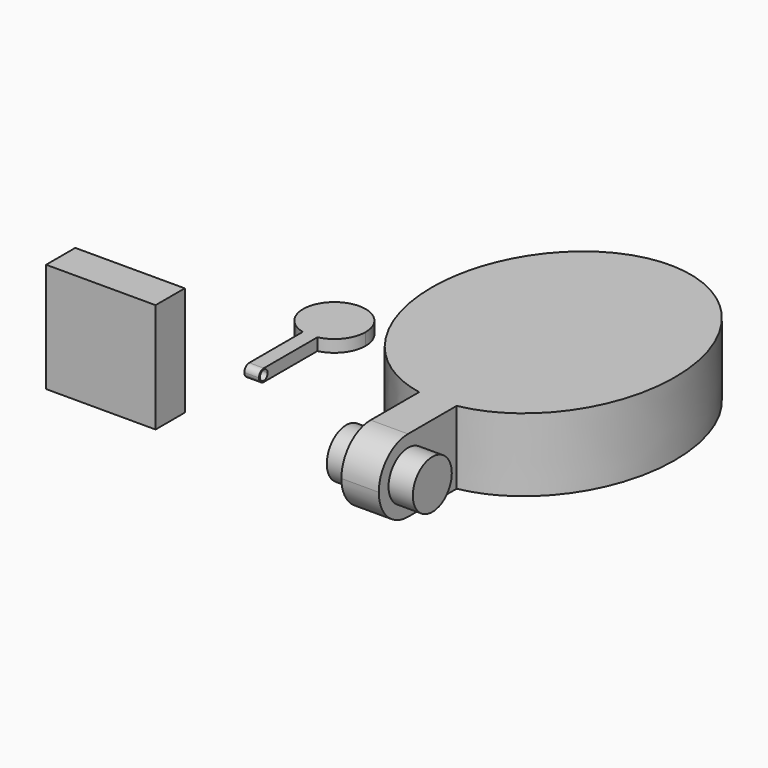
from build123d import *

# Parameters (mm, degrees)
F1_DEPTH  = 5
F2_DEPTH  = 5
F4_DEPTH  = 10
F6_DEPTH  = 5
F8_DEPTH  = 20
F10_DEPTH = 20
F11_R     = 2.5
F12_R     = 2.49999
F13_W     = 6.5
F13_H     = 45
F14_DEPTH = 5
F15_W     = 3
F15_H     = 5
F16_DEPTH = 5
F17_R     = 2
F18_DEPTH = 3
F19_R     = 2
F20_DEPTH = 3
F22_DEPTH = 30
F23_DEPTH = 30
F25_DEPTH = 10
F26_R     = 10
F27_DEPTH = 10
F28_R     = 15
F29_R     = 14.99999


# Not quite as in the source:
# - a fillet or chamfer is up to 0.001 mm smaller than in the source, because OpenCascade refuses the exact size


with BuildPart() as f1:
    # F0 (on Top) → F1 (new body)
    with BuildSketch(Plane.XY):
        with BuildLine():
            ThreePointArc((0, -12.5), (8.8388347648, -8.8388347648), (12.5, 0))
            ThreePointArc((12.5, 0), (-8.8388347648, 8.8388347648), (0, -12.5))
        make_face()
    extrude(amount=F1_DEPTH)

    # F0 (on Top) → F2 (join)
    with BuildSketch(Plane.XY):
        with BuildLine():
            Line((-3, -12.5), (0, -12.5))
            Line((0, -12.5), (3, -12.5))
            ThreePointArc((3, -12.5), (10.0949215053, -7.9588039178), (12.8549601322, 0))
            ThreePointArc((12.8549601322, 0), (-7.9588039178, 10.0949215053), (-3, -12.5))
        make_face()
        with BuildLine():
            ThreePointArc((0, -12.5), (-8.8388347648, 8.8388347648), (12.5, 0))
            ThreePointArc((12.5, 0), (8.8388347648, -8.8388347648), (0, -12.5))
        make_face(mode=Mode.SUBTRACT)
        with BuildLine():
            Line((3, -12.5), (0, -12.5))
            Line((0, -12.5), (-3, -12.5))
            ThreePointArc((-3, -12.5), (0, -12.8549601322), (3, -12.5))
        make_face()
        with BuildLine():
            ThreePointArc((3, -12.5), (0, -12.8549601322), (-3, -12.5))
            Line((-3, -12.5), (-3, -42.5))
            Line((-3, -42.5), (3, -42.5))
            Line((3, -42.5), (3, -12.5))
        make_face()
    extrude(amount=F2_DEPTH)

    # F3 (on face) → F4 (cut)
    with BuildSketch(Plane.YZ.offset(3)):
        with BuildLine():
            ThreePointArc((-40, 4.5), (-41.4142135624, 3.9142135624), (-42, 2.5))
            Line((-42, 2.5), (-40, 2.5))
            Line((-40, 2.5), (-40, 4.5))
        make_face()
        with BuildLine():
            Line((-40, 2.5), (-42, 2.5))
            ThreePointArc((-42, 2.5), (-40, 0.5), (-38, 2.5))
            ThreePointArc((-38, 2.5), (-38.5857864376, 3.9142135624), (-40, 4.5))
            Line((-40, 4.5), (-40, 2.5))
        make_face()
    extrude(amount=-F4_DEPTH, mode=Mode.SUBTRACT)

    # F11
    f11_edges = [f1.edges().sort_by_distance(p)[0] for p in [
        (0, -42.5, 5),
    ]]
    fillet(f11_edges, radius=F11_R)

    # F12 (radius 2.5 in the source; OpenCascade refuses exactly that, so slightly less here)
    f12_edges = [f1.edges().sort_by_distance(p)[0] for p in [
        (0, -42.5, 0),
    ]]
    fillet(f12_edges, radius=F12_R)


with BuildPart() as f6:
    # F5 (on Top) → F6 (new body)
    with BuildSketch(Plane.XY):
        Polygon((-46.75, -47.5), (-50, -47.5), (-53.25, -47.5), (-53.25, -42.5), (-72.5, -42.5), (-72.5, -57.5), (-27.5, -57.5), (-27.5, -42.5), (-46.75, -42.5), align=None)
    extrude(amount=F6_DEPTH)

    # F7 (on face) → F8 (join)
    with BuildSketch(Plane.XY.offset(5)):
        Polygon((-53.25, -42.5), (-72.5, -42.5), (-72.5, -57.5), (-27.5, -57.5), (-27.5, -42.5), (-46.75, -42.5), (-46.75, -47.5), (-53.25, -47.5), align=None)
    extrude(amount=F8_DEPTH)

    # F9 (on face) → F10 (join)
    with BuildSketch(Plane(origin=(0, 0, 0), x_dir=(1, 0, 0), z_dir=(0, 0, -1))):
        Polygon((-46.75, 42.5), (-27.5, 42.5), (-27.5, 57.5), (-72.5, 57.5), (-72.5, 42.5), (-53.25, 42.5), (-53.25, 47.5), (-46.75, 47.5), align=None)
    extrude(amount=F10_DEPTH)

    # F13 (on face) → F14 (join)
    with BuildSketch(Plane(origin=(0, -47.5, 0), x_dir=(-1, 0, 0), z_dir=(0, 1, 0))):
        with Locations((50, 2.5)):
            Rectangle(F13_W, F13_H)
    extrude(amount=F14_DEPTH)

    # F15 (on face) → F16 (join)
    with BuildSketch(Plane(origin=(0, -42.5, 0), x_dir=(-1, 0, 0), z_dir=(0, 1, 0))):
        with Locations((54.5, 2.5)):
            Rectangle(F15_W, F15_H)
        with Locations((45.5, 2.5)):
            Rectangle(F15_W, F15_H)
    extrude(amount=F16_DEPTH)

    # F17 (on face) → F18 (cut)
    with BuildSketch(Plane(origin=(-56, 0, 0), x_dir=(0, -1, 0), z_dir=(-1, 0, 0))):
        with Locations((40, 2.5)):
            Circle(F17_R)
    extrude(amount=-F18_DEPTH, mode=Mode.SUBTRACT)

    # F19 (on face) → F20 (cut)
    with BuildSketch(Plane.YZ.offset(-44)):
        with Locations((-40, 2.5)):
            Circle(F19_R)
    extrude(amount=-F20_DEPTH, mode=Mode.SUBTRACT)


with BuildPart() as f22:
    # F21 (on Top) → F22 (new body)
    with BuildSketch(Plane.XY):
        with BuildLine():
            add(Edge.make_bspline(
                [(90, -60), (93.8671431109, -60), (97.6882954661, -59.2864382677)],
                knots=[0, 0, 0, 0.1543783876, 0.1543783876, 0.1543783876], degree=2, weights=[1, 0.997022393, 1]))
            Line((97.6882954661, -59.2864382677), (90, -59.2864382677))
            Line((90, -59.2864382677), (90, -60))
        make_face()
        with BuildLine():
            add(Edge.make_bspline(
                [(97.6882954661, -59.2864382677), (205.0474477085, -39.2381974411), (122.5237238542, 45.5716867888), (40, 130.3815710188), (40, 0)],
                knots=[0.1543783876, 0.1543783876, 0.1543783876, 2.433383684, 2.433383684, 4.7123889804, 4.7123889804, 4.7123889804], degree=2, weights=[1, 0.4180463628, 1, 0.4180463628, 1]))
            Line((40, 0), (90, 0))
            Line((90, 0), (90, -59.2864382677))
            Line((90, -59.2864382677), (97.6882954661, -59.2864382677))
        make_face()
        with BuildLine():
            Line((90, 0), (40, 0))
            add(Edge.make_bspline(
                [(40, 0), (40, -51.3851534255), (82.3117045339, -59.2864382677)],
                knots=[4.7123889804, 4.7123889804, 4.7123889804, 6.1288069195, 6.1288069195, 6.1288069195], degree=2, weights=[1, 0.7595281131, 1]))
            Line((82.3117045339, -59.2864382677), (90, -59.2864382677))
            Line((90, -59.2864382677), (90, 0))
        make_face()
        with BuildLine():
            Line((90, -59.2864382677), (82.3117045339, -59.2864382677))
            add(Edge.make_bspline(
                [(82.3117045339, -59.2864382677), (86.1328568891, -60), (90, -60)],
                knots=[6.1288069195, 6.1288069195, 6.1288069195, 6.2831853072, 6.2831853072, 6.2831853072], degree=2, weights=[1, 0.997022393, 1]))
            Line((90, -60), (90, -59.2864382677))
        make_face()
    extrude(amount=F22_DEPTH)

    # F21 (on Top) → F23 (join)
    with BuildSketch(Plane.XY):
        with BuildLine():
            add(Edge.make_bspline(
                [(97.6882954661, -59.2864382677), (205.0474477085, -39.2381974411), (122.5237238542, 45.5716867888), (40, 130.3815710188), (40, 0)],
                knots=[0.1543783876, 0.1543783876, 0.1543783876, 2.433383684, 2.433383684, 4.7123889804, 4.7123889804, 4.7123889804], degree=2, weights=[1, 0.4180463628, 1, 0.4180463628, 1]))
            Line((40, 0), (90, 0))
            Line((90, 0), (90, -59.2864382677))
            Line((90, -59.2864382677), (97.6882954661, -59.2864382677))
        make_face()
        with BuildLine():
            Line((90, 0), (40, 0))
            add(Edge.make_bspline(
                [(40, 0), (40, -51.3851534255), (82.3117045339, -59.2864382677)],
                knots=[4.7123889804, 4.7123889804, 4.7123889804, 6.1288069195, 6.1288069195, 6.1288069195], degree=2, weights=[1, 0.7595281131, 1]))
            Line((82.3117045339, -59.2864382677), (90, -59.2864382677))
            Line((90, -59.2864382677), (90, 0))
        make_face()
        with BuildLine():
            Line((97.6882954661, -99.2864382677), (97.6882954661, -59.2864382677))
            add(Edge.make_bspline(
                [(90, -60), (93.8671431109, -60), (97.6882954661, -59.2864382677)],
                knots=[0, 0, 0, 0.1543783876, 0.1543783876, 0.1543783876], degree=2, weights=[1, 0.997022393, 1]))
            add(Edge.make_bspline(
                [(82.3117045339, -59.2864382677), (86.1328568891, -60), (90, -60)],
                knots=[6.1288069195, 6.1288069195, 6.1288069195, 6.2831853072, 6.2831853072, 6.2831853072], degree=2, weights=[1, 0.997022393, 1]))
            Line((82.3117045339, -59.2864382677), (82.3117045339, -99.2864382677))
            Line((82.3117045339, -99.2864382677), (97.6882954661, -99.2864382677))
        make_face()
        with BuildLine():
            add(Edge.make_bspline(
                [(90, -60), (93.8671431109, -60), (97.6882954661, -59.2864382677)],
                knots=[0, 0, 0, 0.1543783876, 0.1543783876, 0.1543783876], degree=2, weights=[1, 0.997022393, 1]))
            Line((97.6882954661, -59.2864382677), (90, -59.2864382677))
            Line((90, -59.2864382677), (90, -60))
        make_face()
        with BuildLine():
            Line((90, -59.2864382677), (82.3117045339, -59.2864382677))
            add(Edge.make_bspline(
                [(82.3117045339, -59.2864382677), (86.1328568891, -60), (90, -60)],
                knots=[6.1288069195, 6.1288069195, 6.1288069195, 6.2831853072, 6.2831853072, 6.2831853072], degree=2, weights=[1, 0.997022393, 1]))
            Line((90, -60), (90, -59.2864382677))
        make_face()
    extrude(amount=F23_DEPTH)

    # F24 (on face) → F25 (join)
    with BuildSketch(Plane.YZ.offset(97.6882954661)):
        with BuildLine():
            ThreePointArc((-94.2864382677, 15), (-84.2864382677, 5), (-74.2864382677, 15))
            ThreePointArc((-74.2864382677, 15), (-84.2864382677, 25), (-94.2864382677, 15))
        make_face()
    extrude(amount=F25_DEPTH)

    # F26 (on face) → F27 (join)
    with BuildSketch(Plane(origin=(82.3117045339, 0, 0), x_dir=(0, -1, 0), z_dir=(-1, 0, 0))):
        with Locations((84.2864382677, 15)):
            Circle(F26_R)
    extrude(amount=F27_DEPTH)

    # F28
    f28_edges = [f22.edges().sort_by_distance(p)[0] for p in [
        (90, -99.286438, 30),
    ]]
    fillet(f28_edges, radius=F28_R)

    # F29 (radius 15 in the source; OpenCascade refuses exactly that, so slightly less here)
    f29_edges = [f22.edges().sort_by_distance(p)[0] for p in [
        (90, -99.286438, 0),
    ]]
    fillet(f29_edges, radius=F29_R)


solid = Compound([f1.part, f6.part, f22.part])
